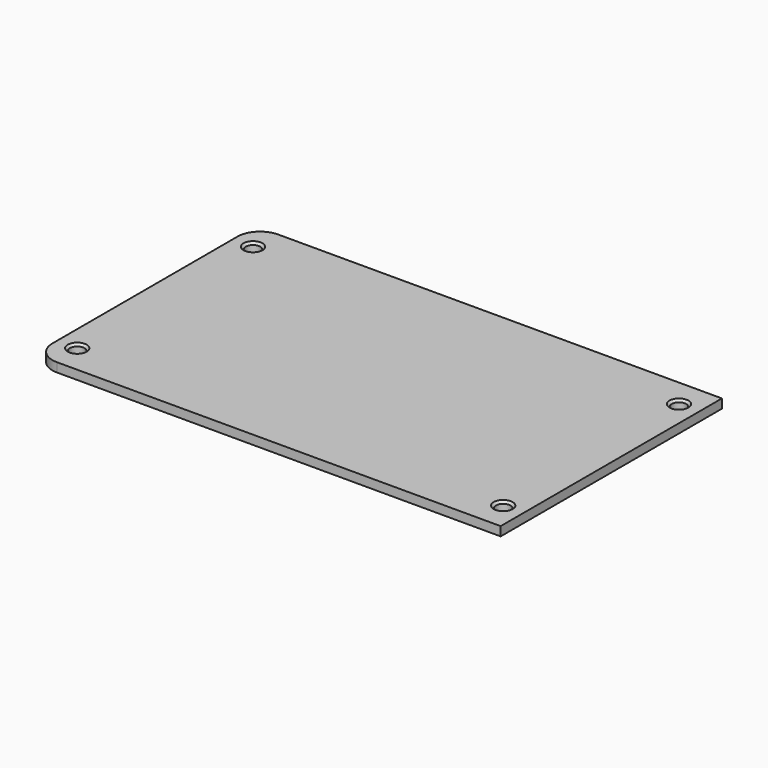
from build123d import *

# Parameters (mm, degrees)
F0_W     = 103.0236035585
F0_H     = 61.1
F0_R     = 1.6
F1_DEPTH = 2
F2_R     = 5
F3_SIZE  = 0.5


with BuildPart() as f1:
    # F0 (on Top) → F1 (new body)
    with BuildSketch(Plane.XY):
        Rectangle(F0_W, F0_H)
        with Locations((-47.05, -24.27)):
            Circle(F0_R, mode=Mode.SUBTRACT)
        with BuildLine():
            ThreePointArc((45.45, -24.27), (47.05, -22.67), (48.65, -24.27))
            ThreePointArc((48.65, -24.27), (47.05, -25.87), (45.45, -24.27))
        make_face(mode=Mode.SUBTRACT)
        with Locations((-47.05, 24.27)):
            Circle(F0_R, mode=Mode.SUBTRACT)
        with Locations((47.05, 24.27)):
            Circle(F0_R, mode=Mode.SUBTRACT)
    extrude(amount=F1_DEPTH)

    # F2
    f2_edges = [f1.edges().sort_by_distance(p)[0] for p in [
        (-51.511802, -30.55, 1),
        (-51.511802, 30.55, 1),
    ]]
    fillet(f2_edges, radius=F2_R)

    # F3
    f3_edges = [f1.edges().sort_by_distance(p)[0] for p in [
        (-48.65, -24.27, 2),
        (-48.65, 24.27, 2),
        (45.45, 24.27, 2),
        (48.65, -24.27, 2),
    ]]
    chamfer(f3_edges, length=F3_SIZE)


solid = f1.part
